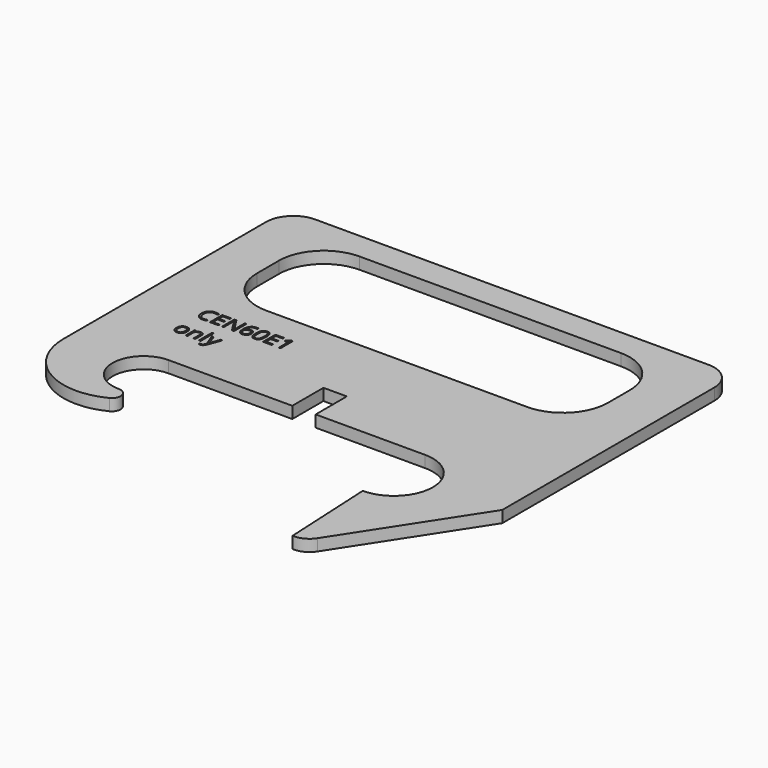
from build123d import *

# Parameters (mm, degrees)
F1_DEPTH     = 3
F2_TEXT_SIZE = 5.5555555556
F3_DEPTH     = 1


# Not quite as in the source:
# - Text() gives the source's letters only with a copy of the font that has no kerning and outlines rounded to 1/6400 em; it was checked with that copy


with BuildPart() as f1:
    # F0 (on Top) → F1 (new body)
    with BuildSketch(Plane.XY):
        with BuildLine():
            Line((-31.7111682197, 0), (0, 0))
            Line((0, 0), (0, 10))
            Line((0, 10), (6, 10))
            Line((6, 10), (6, 0))
            Line((6, 0), (34.08, 0))
            ThreePointArc((34.08, 0), (44.08, -10), (34.08, -20))
            Line((34.08, -20), (35.28, -44))
            ThreePointArc((35.28, -44), (37.8593830481, -43.4866448347), (39.8214309088, -41.7353257243))
            Line((39.8214309088, -41.7353257243), (61.08, -9))
            Line((61.08, -9), (61.08, 59))
            ThreePointArc((61.08, 59), (59.0297474683, 63.9497474683), (54.08, 66))
            Line((54.08, 66), (-46.92, 66))
            ThreePointArc((-46.92, 66), (-51.8697474683, 63.9497474683), (-53.92, 59))
            Line((-53.92, 59), (-53.92, -5.9629004314))
            ThreePointArc((-53.92, -5.9629004314), (-46.3008425214, -19.5923347055), (-30.699815171, -20.2411682197))
            ThreePointArc((-30.699815171, -20.2411682197), (-29.5311256251, -17.721313168), (-31.7111682197, -16))
            ThreePointArc((-31.7111682197, -16), (-39.7111682197, -8), (-31.7111682197, 0))
        make_face()
        with BuildLine():
            ThreePointArc((-41.42, 47.5180073699), (-38.0570022202, 55.6370022202), (-29.9380073699, 59))
            Line((-29.9380073699, 59), (37.0980073699, 59))
            ThreePointArc((37.0980073699, 59), (45.2170022202, 55.6370022202), (48.58, 47.5180073699))
            Line((48.58, 47.5180073699), (48.58, 40.4819926301))
            ThreePointArc((48.58, 40.4819926301), (45.2170022202, 32.3629977798), (37.0980073699, 29))
            Line((37.0980073699, 29), (-29.9380073699, 29))
            ThreePointArc((-29.9380073699, 29), (-38.0570022202, 32.3629977798), (-41.42, 40.4819926301))
            Line((-41.42, 40.4819926301), (-41.42, 47.5180073699))
        make_face(mode=Mode.SUBTRACT)
    extrude(amount=F1_DEPTH)

    # F2 (on face) → F3 (cut)
    with BuildSketch(Plane.XY.offset(3)):
        with Locations((-39.5885637254, 18.0181560689)):
            Text('CEN60E1', F2_TEXT_SIZE, font='Open Sans', text_align=(TextAlign.LEFT, TextAlign.BOTTOM))
        with Locations((-39.5885637254, 10.4626005134)):
            Text('only', F2_TEXT_SIZE, font='Open Sans', text_align=(TextAlign.LEFT, TextAlign.BOTTOM))
    extrude(amount=-F3_DEPTH, mode=Mode.SUBTRACT)


solid = f1.part
